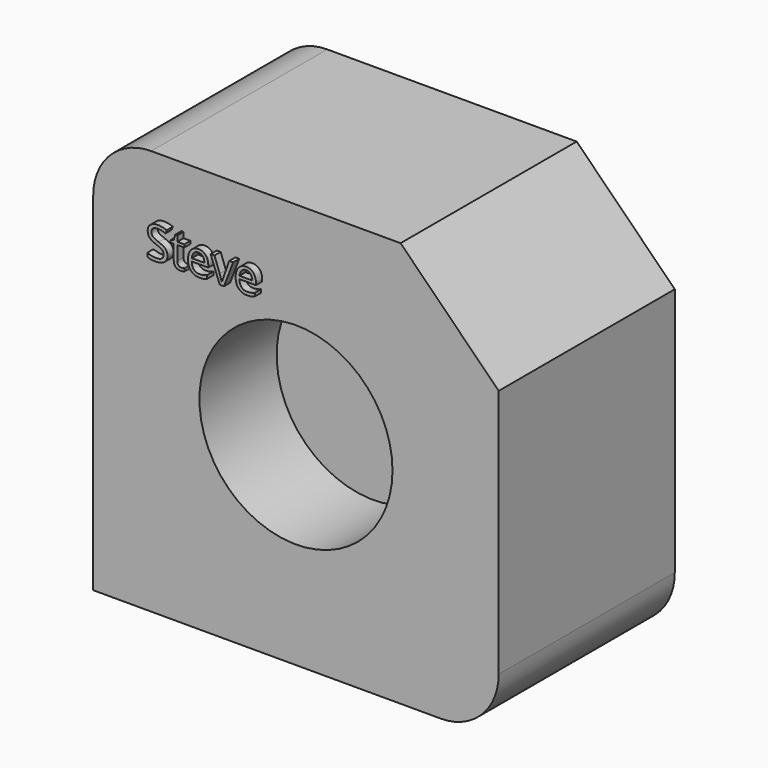
from build123d import *

# Parameters (mm, degrees)
F1_DEPTH     = 57
F2_R         = 25
F3_DEPTH     = 25
F4_TEXT_SIZE = 11.6203998023
F5_DEPTH     = 2


# Not quite as in the source:
# - Text() gives the source's letters only with a copy of the font that has no kerning and outlines rounded to 1/6400 em; it was checked with that copy


with BuildPart() as f1:
    # F0 (on Front) → F1 (new body)
    with BuildSketch(Plane.XZ):
        with BuildLine():
            Line((30.7267345488, 50.2887536223), (-33.8662554746, 50.2887536223))
            ThreePointArc((-33.8662554746, 50.2887536223), (-44.4728571924, 45.8953553401), (-48.8662554746, 35.2887536223))
            Line((-48.8662554746, 35.2887536223), (-48.8662554746, -54.7112463777))
            Line((-48.8662554746, -54.7112463777), (41.1337445254, -54.7112463777))
            ThreePointArc((41.1337445254, -54.7112463777), (51.7403462432, -50.3178480955), (56.1337445254, -39.7112463777))
            Line((56.1337445254, -39.7112463777), (56.1337445254, 24.8817436457))
            Line((56.1337445254, 24.8817436457), (30.7267345488, 50.2887536223))
        make_face()
    extrude(amount=F1_DEPTH)

    # F2 (on face) → F3 (cut)
    with BuildSketch(Plane.XZ.offset(57)):
        with Locations((3.6337445254, -2.2112463777)):
            Circle(F2_R)
    extrude(amount=-F3_DEPTH, mode=Mode.SUBTRACT)

    # F4 (on face) → F5 (join)
    with BuildSketch(Plane.XZ.offset(57)):
        with Locations((-33.8662554746, 26.9220657647)):
            Text('Steve', F4_TEXT_SIZE, font='Open Sans', text_align=(TextAlign.LEFT, TextAlign.BOTTOM))
    extrude(amount=F5_DEPTH)


solid = f1.part
